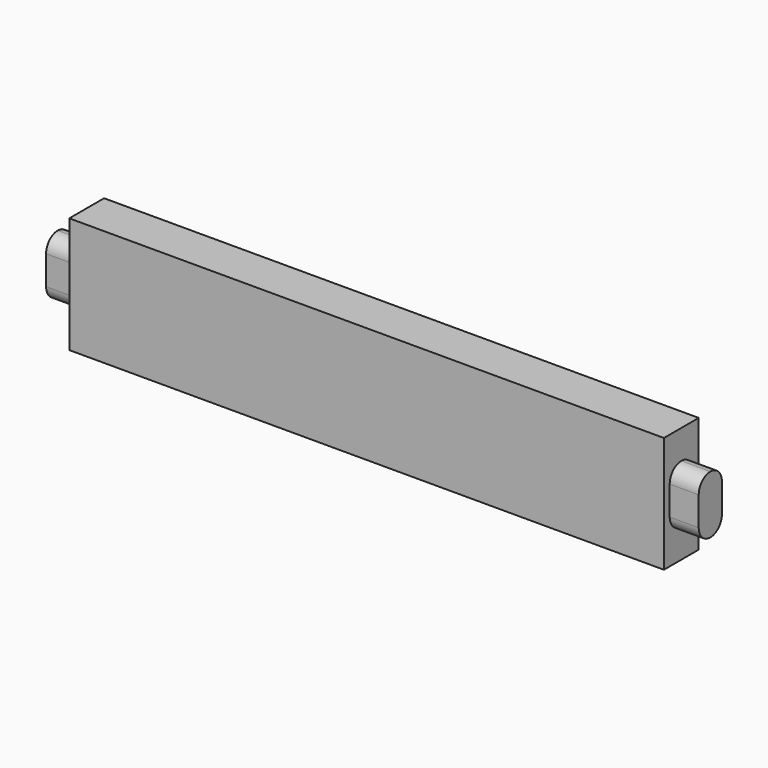
from build123d import *

# Parameters (mm, degrees)
F0_W     = 260.35
F0_H     = 19.05
F1_DEPTH = 50.8
F2_W     = 12.7
F2_H     = 25.4
F3_DEPTH = 12.7
F4_R     = 6.34999
F5_W     = 12.7
F5_H     = 25.4
F6_DEPTH = 12.7
F7_R     = 6.34999


# Not quite as in the source:
# - a fillet or chamfer is up to 0.001 mm smaller than in the source, because OpenCascade refuses the exact size


with BuildPart() as f1:
    # F0 (on Top) → F1 (new body)
    with BuildSketch(Plane.XY):
        Rectangle(F0_W, F0_H)
    extrude(amount=-F1_DEPTH)

    # F2 (on face) → F3 (join)
    with BuildSketch(Plane(origin=(-130.175, 0, 0), x_dir=(0, -1, 0), z_dir=(-1, 0, 0))):
        with Locations((0, -25.4)):
            Rectangle(F2_W, F2_H)
    extrude(amount=F3_DEPTH)

    # F4 (radius 6.35 in the source; OpenCascade refuses exactly that, so slightly less here)
    f4_edges = [f1.edges().sort_by_distance(p)[0] for p in [
        (-136.525, 6.35, -12.7),
        (-136.525, -6.35, -12.7),
        (-136.525, -6.35, -38.1),
        (-136.525, 6.35, -38.1),
    ]]
    fillet(f4_edges, radius=F4_R)

    # F5 (on face) → F6 (join)
    with BuildSketch(Plane.YZ.offset(130.175)):
        with Locations((0, -25.4)):
            Rectangle(F5_W, F5_H)
    extrude(amount=F6_DEPTH)

    # F7 (radius 6.35 in the source; OpenCascade refuses exactly that, so slightly less here)
    f7_edges = [f1.edges().sort_by_distance(p)[0] for p in [
        (136.525, -6.35, -12.7),
        (136.525, 6.35, -12.7),
        (136.525, 6.35, -38.1),
        (136.525, -6.35, -38.1),
    ]]
    fillet(f7_edges, radius=F7_R)


solid = f1.part
